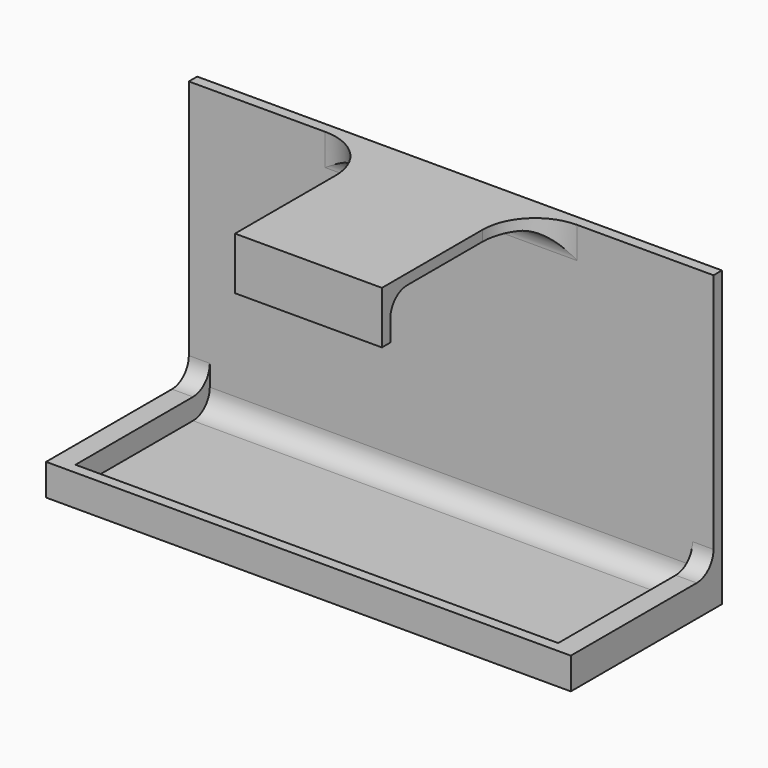
from build123d import *

# Parameters (mm, degrees)
F1_DEPTH = 50
F2_W     = 2
F2_H     = 16
F3_DEPTH = 2
F4_W     = 18
F4_H     = 17
F5_DEPTH = 25
F7_R     = 5
F8_R     = 1.9999


# Not quite as in the source:
# - a fillet or chamfer is up to 0.001 mm smaller than in the source, because OpenCascade refuses the exact size
# - a feature of the source that left no trace in its solid (it failed there, or was rolled back) is left out


with BuildPart() as f1:
    # F0 (on Right) → F1 (new body)
    with BuildSketch(Plane.YZ):
        Polygon((0, 26), (0, 0), (-16, 0), (-16, 2), (-17, 2), (-17, -1), (1, -1), (1, 26), align=None)
        Polygon((-16, 26), (0, 26), (1, 26), (1, 27), (-17, 27), (-17, 22), (-16, 22), align=None)
    extrude(amount=F1_DEPTH)

    # F2 (on face) → F3 (join)
    with BuildSketch(Plane.XY):
        with Locations((1, -8)):
            Rectangle(F2_W, F2_H)
        with Locations((49, -8)):
            Rectangle(F2_W, F2_H)
    extrude(amount=F3_DEPTH)

    # F4 (on face) → F5 (cut)
    with BuildSketch(Plane.XY.offset(27)):
        with Locations((9, -8.5)):
            Rectangle(F4_W, F4_H)
        with Locations((41, -8.5)):
            Rectangle(F4_W, F4_H)
    extrude(amount=-F5_DEPTH, mode=Mode.SUBTRACT)

    # F7
    f7_edges = [f1.edges().sort_by_distance(p)[0] for p in [
        (32, 0, 26.5),
        (18, 0, 26.5),
    ]]
    fillet(f7_edges, radius=F7_R)

    # F8 (radius 2 in the source; OpenCascade refuses exactly that, so slightly less here)
    f8_edges = [f1.edges().sort_by_distance(p)[0] for p in [
        (25, -16, 0),
        (1, 0, 2),
        (25, 0, 26),
        (25, 0, 0),
        (49, 0, 2),
        (25, -16, 26),
    ]]
    fillet(f8_edges, radius=F8_R)


solid = f1.part
